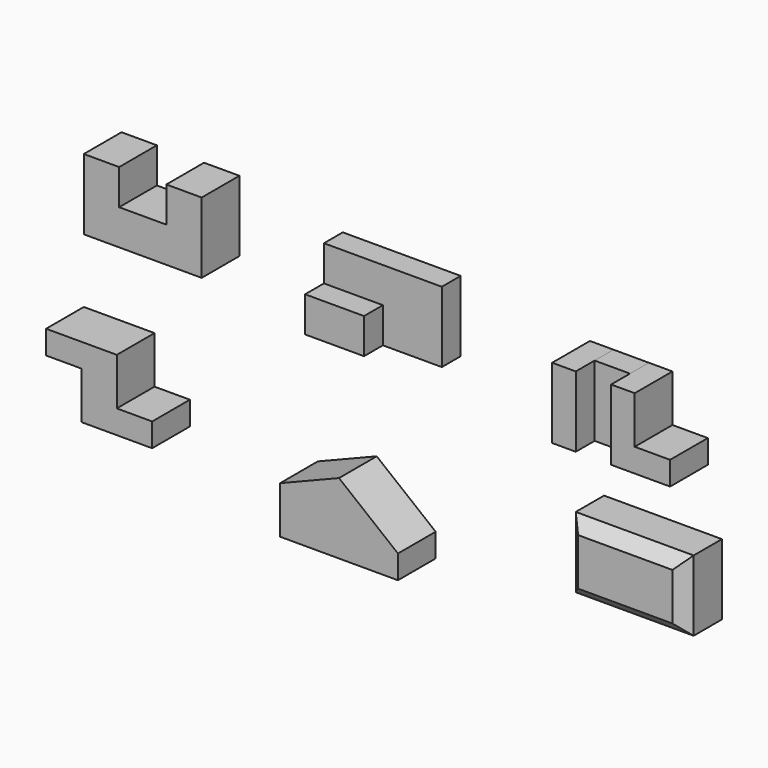
from build123d import *

# Parameters (mm, degrees)
F1_DEPTH  = 101.6
F2_W      = 127
F2_H      = 76.2
F3_DEPTH  = 50.8
F4_W      = 127
F4_H      = 76.2
F5_DEPTH  = 50.8
F7_DEPTH  = 101.6
F6_W      = 50.8
F6_H      = 152.4
F8_W      = 76.2
F8_H      = 152.4
F9_DEPTH  = 50.8
F11_DEPTH = 101.6
F13_W     = 254
F13_H     = 152.4
F14_DEPTH = 101.6
F15_DEPTH = 101.6
F16_SIZE  = 25.4


# Not quite as in the source:
# - a feature names something its author has since deleted; it is built from what else it names


with BuildPart() as f1:
    # F0 (on Front) → F1 (new body)
    with BuildSketch(Plane.XZ):
        Polygon((0, 152.4), (0, 0), (254, 0), (254, 152.4), (177.8, 152.4), (177.8, 76.2), (76.2, 76.2), (76.2, 152.4), align=None)
    extrude(amount=-F1_DEPTH)


with BuildPart() as f3:
    # F2 (on Front) → F3 (new body)
    with BuildSketch(Plane.XZ):
        with Locations((580.9306057492, 37.1004903008)):
            Rectangle(F2_W, F2_H)
    extrude(amount=F3_DEPTH)

    # F4 (on face) → F5 (join)
    with BuildSketch(Plane(origin=(0, 0, 0), x_dir=(-1, 0, 0), z_dir=(0, 1, 0))):
        with Locations((-580.9306057492, 37.1004903008)):
            Rectangle(F4_W, F4_H)
        Polygon((-771.4306057492, -0.9995096992), (-644.4306057492, -0.9995096992), (-644.4306057492, 75.2004903008), (-517.4306057492, 75.2004903008), (-517.4306057492, 151.4004903008), (-771.4306057492, 151.4004903008), align=None)
    extrude(amount=F5_DEPTH)


with BuildPart() as f7:
    # F6 (on face) → F7 (new body)
    with BuildSketch(Plane.XZ):
        Polygon((1268.3531419389, 152.4), (1217.5531419389, 152.4), (1217.5531419389, 0), (1344.5531419389, 0), (1344.5531419389, 50.8), (1268.3531419389, 50.8), align=None)
    extrude(amount=F7_DEPTH)


with BuildPart() as f7b:
    # F6 (on face) → F7, piece 2 (new body)
    with BuildSketch(Plane.XZ):
        with Locations((1115.9531419389, 76.2)):
            Rectangle(F6_W, F6_H)
    extrude(amount=F7_DEPTH)


with BuildPart() as f9:
    # F8 (on face) → F9 (new body)
    with BuildSketch(Plane(origin=(0, 0, 0), x_dir=(-1, 0, 0), z_dir=(0, 1, 0))):
        with Locations((-1179.4531419389, 76.2)):
            Rectangle(F8_W, F8_H)
    extrude(amount=-F9_DEPTH)


with BuildPart() as f11:
    # F10 (on face) → F11 (new body)
    with BuildSketch(Plane.XZ):
        Polygon((152.4, -137.7568855792), (0, -137.7568855792), (0, -188.5568855792), (76.2, -188.5568855792), (76.2, -290.1568855792), (228.6, -290.1568855792), (228.6, -239.3568855792), (152.4, -239.3568855792), align=None)
    extrude(amount=F11_DEPTH)


with BuildPart() as f14:
    # F13 (on face) → F14 (new body)
    with BuildSketch(Plane.XZ):
        with Locations((1247.9882836342, -207.20400113)):
            Rectangle(F13_W, F13_H)
    extrude(amount=F14_DEPTH)

    # F16
    f16_edges = [f14.edges().sort_by_distance(p)[0] for p in [
        (1247.988284, -101.6, -131.004001),
        (1374.988284, -101.6, -207.204001),
        (1247.988284, -101.6, -283.404001),
        (1120.988284, -101.6, -207.204001),
    ]]
    chamfer(f16_edges, length=F16_SIZE)


with BuildPart() as f15:
    # F12 (on face) → F15 (new body)
    with BuildSketch(Plane.XZ.offset(101.6)):
        Polygon((585.472053026, -199.0268103926), (585.472053026, -300.6268103926), (839.472053026, -300.6268103926), (839.472053026, -249.8268103926), (712.472053026, -148.0449278362), align=None)
    extrude(amount=F15_DEPTH)


solid = Compound([f1.part, f3.part, f7.part, f7b.part, f9.part, f11.part, f14.part, f15.part])
